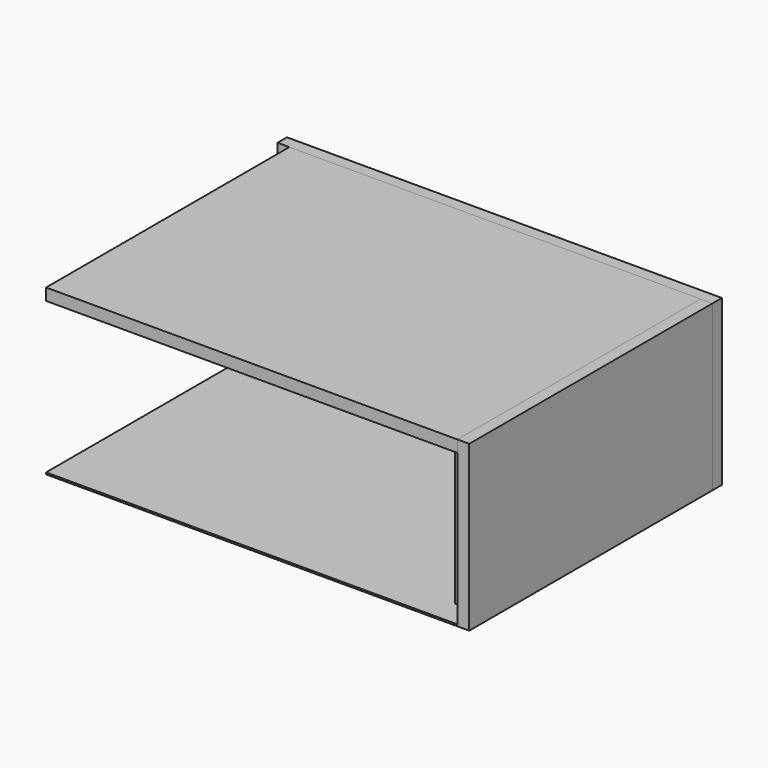
from build123d import *

# Parameters (mm, degrees)
F0_W      = 230
F0_H      = 170
F1_DEPTH  = 1
F2_W      = 170
F2_H      = 92
F3_DEPTH  = 6.6
F4_W      = 243.2
F4_H      = 92
F5_DEPTH  = 6.6
F6_W      = 230
F6_H      = 79
F7_DEPTH  = 6.6
F8_W      = 156.8
F8_H      = 79
F9_DEPTH  = 6.6
F10_W     = 230
F10_H     = 170
F11_DEPTH = 6.6


# Not quite as in the source:
# - a feature names something its author has since deleted; it is built from what else it names


with BuildPart() as f1:
    # F0 (on Top) → F1 (new body)
    with BuildSketch(Plane.XY):
        Rectangle(F0_W, F0_H)
    extrude(amount=F1_DEPTH)


with BuildPart() as f3:
    # F2 (on face) → F3 (new body)
    with BuildSketch(Plane.YZ.offset(115)):
        with Locations((0, 46)):
            Rectangle(F2_W, F2_H)
    extrude(amount=F3_DEPTH)


with BuildPart() as f5:
    # F4 (on face) → F5 (new body)
    with BuildSketch(Plane(origin=(0, 85, 0), x_dir=(-1, 0, 0), z_dir=(0, 1, 0))):
        with Locations((0, 46)):
            Rectangle(F4_W, F4_H)
    extrude(amount=F5_DEPTH)


with BuildPart() as f7:
    # F6 (on face) → F7 (new body)
    with BuildSketch(Plane.XZ.offset(-85)):
        with Locations((0, 45.9)):
            Rectangle(F6_W, F6_H)
    extrude(amount=F7_DEPTH)


with BuildPart() as f9:
    # F8 (on face) → F9 (new body)
    with BuildSketch(Plane(origin=(115, 0, 0), x_dir=(0, -1, 0), z_dir=(-1, 0, 0))):
        with Locations((0, 45.9)):
            Rectangle(F8_W, F8_H)
    extrude(amount=F9_DEPTH)


with BuildPart() as f11:
    # F10 (on face) → F11 (new body)
    with BuildSketch(Plane.XY.offset(85.4)):
        Rectangle(F10_W, F10_H)
    extrude(amount=F11_DEPTH)


solid = Compound([f1.part, f3.part, f5.part, f7.part, f9.part, f11.part])
